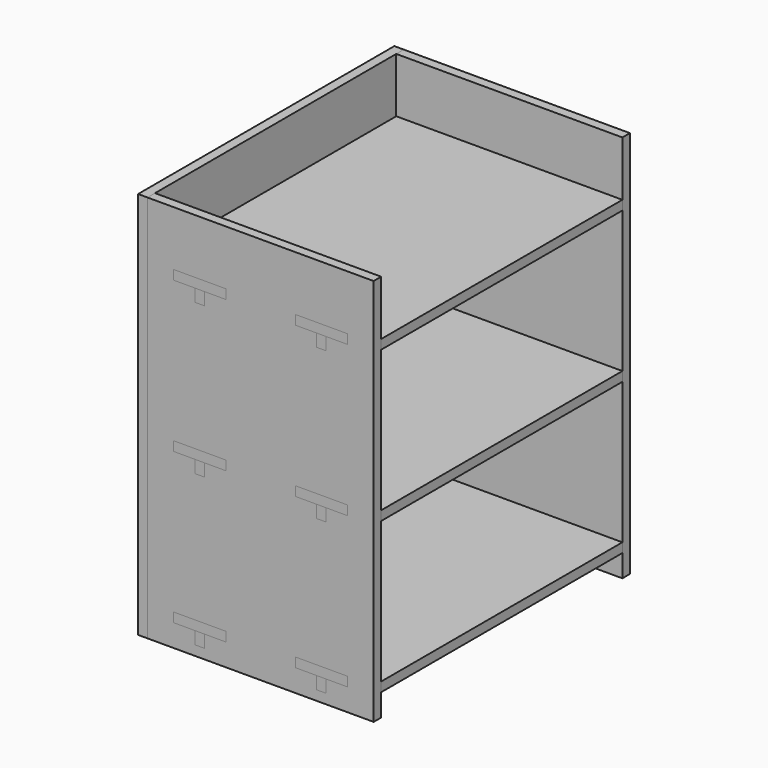
from build123d import *

# Parameters (mm, degrees)
F2_DEPTH  = 19.05
F3_W      = 19.05
F3_H      = 25.4
F4_DEPTH  = 647.7
F5_W      = 19.05
F5_H      = 7.62
F6_DEPTH  = 609.6
F9_W      = 457.2
F9_H      = 784.6937250656
F9_W_2    = 140.3600632475
F9_H_2    = 19.05
F10_DEPTH = 19.05
F13_W     = 628.65
F13_H     = 784.6937250656
F13_W_2   = 19.05
F14_DEPTH = 19.05


# Not quite as in the source:
# - a variable given as a bare number and used for a length is read in inches; the dataset says mm whatever the document's units were


with BuildPart() as f2:
    # F1 (on Top) → F2 (new body)
    with BuildSketch(Plane.XY):
        Polygon((356.1228869517, -304.8), (356.1228869517, 0), (356.1228869517, 304.8), (303.1109332372, 304.8), (303.1109332372, 323.85), (197.7029185755, 323.85), (197.7029185755, 304.8), (57.342855328, 304.8), (57.342855328, 323.85), (-48.0651593338, 323.85), (-48.0651593338, 304.8), (-101.0771130483, 304.8), (-101.0771130483, 208.2908415894), (-120.1271130483, 208.2908415894), (-120.1271130483, 96.5091584106), (-101.0771130483, 96.5091584106), (-101.0771130483, 0), (-101.0771130483, -96.5091584106), (-120.1271130483, -96.5091584106), (-120.1271130483, -208.2908415894), (-101.0771130483, -208.2908415894), (-101.0771130483, -304.8), (-48.0651593338, -304.8), (-48.0651593338, -323.85), (57.342855328, -323.85), (57.342855328, -304.8), (197.7029185755, -304.8), (197.7029185755, -323.85), (303.1109332372, -323.85), (303.1109332372, -304.8), align=None)
    extrude(amount=F2_DEPTH)


with BuildPart() as f4:
    # F3 (on face) → F4 (new body, through all)
    with BuildSketch(Plane(origin=(0, 323.85, 0), x_dir=(-1, 0, 0), z_dir=(0, 1, 0))):
        with Locations((-250.4069259064, -12.7)):
            Rectangle(F3_W, F3_H)
    extrude(amount=-F4_DEPTH)

    # F5 (on face) → F6 (join, through all)
    with BuildSketch(Plane(origin=(0, 304.8, 0), x_dir=(-1, 0, 0), z_dir=(0, 1, 0))):
        with Locations((-250.4069259064, -29.21)):
            Rectangle(F5_W, F5_H)
    extrude(amount=-F6_DEPTH)


with BuildPart() as f4b:
    # F3 (on face) → F4, piece 2 (new body, through all)
    with BuildSketch(Plane(origin=(0, 323.85, 0), x_dir=(-1, 0, 0), z_dir=(0, 1, 0))):
        with Locations((-4.6388479971, -12.7)):
            Rectangle(F3_W, F3_H)
    extrude(amount=-F4_DEPTH)

    # F5 (on face) → F6, piece 2 (join, through all)
    with BuildSketch(Plane(origin=(0, 304.8, 0), x_dir=(-1, 0, 0), z_dir=(0, 1, 0))):
        with Locations((-4.6388479971, -29.21)):
            Rectangle(F5_W, F5_H)
    extrude(amount=-F6_DEPTH)


with BuildPart() as f7_1:
    # F7: copy of F2
    add(f2.part.moved(Location((0, 0, -304.8))))


with BuildPart() as f7_2:
    # F7: copy of F4
    add(f4.part.moved(Location((0, 0, -304.8))))


with BuildPart() as f7_3:
    # F7: copy of F4b
    add(f4b.part.moved(Location((0, 0, -304.8))))


with BuildPart() as f8_1:
    # F8: copy of F7_1
    add(f7_1.part.moved(Location((0, 0, -304.8))))


with BuildPart() as f8_2:
    # F8: copy of F7_2
    add(f7_2.part.moved(Location((0, 0, -304.8))))


with BuildPart() as f8_3:
    # F8: copy of F7_3
    add(f7_3.part.moved(Location((0, 0, -304.8))))


with BuildPart() as f10:
    # F9 (on face) → F10 (new body)
    with BuildSketch(Plane.XZ.offset(304.8)):
        with Locations((127.5228869517, -262.3551554448)):
            Rectangle(F9_W, F9_H)
        with Locations((127.5228869517, 9.525)):
            Rectangle(F9_W_2, F9_H_2, mode=Mode.SUBTRACT)
        with Locations((127.5228869517, 9.525)):
            Rectangle(F9_W_2, F9_H_2)
    extrude(amount=F10_DEPTH)

    # F11: cut F2, F7_1, F8_1, F4b, F4, F7_3, F7_2, F8_3, F8_2
    add(f2.part, mode=Mode.SUBTRACT)
    add(f7_1.part, mode=Mode.SUBTRACT)
    add(f8_1.part, mode=Mode.SUBTRACT)
    add(f4b.part, mode=Mode.SUBTRACT)
    add(f4.part, mode=Mode.SUBTRACT)
    add(f7_3.part, mode=Mode.SUBTRACT)
    add(f7_2.part, mode=Mode.SUBTRACT)
    add(f8_3.part, mode=Mode.SUBTRACT)
    add(f8_2.part, mode=Mode.SUBTRACT)


with BuildPart() as f12_1:
    # F12: instance of F10
    add(f10.part.mirror(Plane.XZ))


with BuildPart() as f14:
    # F13 (on face) → F14 (new body)
    with BuildSketch(Plane(origin=(-101.0771130483, 0, 0), x_dir=(0, -1, 0), z_dir=(-1, 0, 0))):
        with Locations((9.525, -262.3551554448)):
            Rectangle(F13_W, F13_H)
        with Locations((-314.325, -262.3551554448)):
            Rectangle(F13_W_2, F13_H)
    extrude(amount=F14_DEPTH)

    # F15: cut F2, F7_1, F8_1
    add(f2.part, mode=Mode.SUBTRACT)
    add(f7_1.part, mode=Mode.SUBTRACT)
    add(f8_1.part, mode=Mode.SUBTRACT)


solid = Compound([f2.part, f4.part, f4b.part, f7_1.part, f7_2.part, f7_3.part, f8_1.part, f8_2.part, f8_3.part, f10.part, f12_1.part, f14.part])
